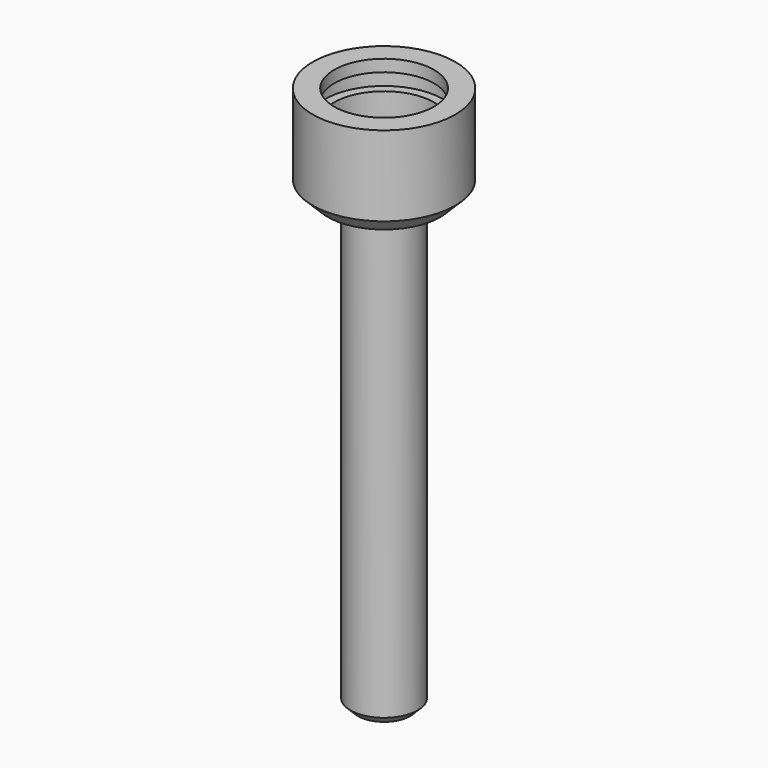
from build123d import *

# Parameters (mm, degrees)
F0_R     = 9.525
F1_DEPTH = 12.7
F2_R     = 6.6675
F3_DEPTH = 9.525
F4_W     = 1.1938
F4_H     = 2.2352
F7_SIZE  = 2
F8_R     = 4.485
F9_DEPTH = 60
F10_SIZE = 1


# Not quite as in the source:
# - the program builds the solid bodies; features that only make, move or delete a surface that nothing else refers to are left out


with BuildPart() as f1:
    # F0 (on Top) → F1 (new body)
    with BuildSketch(Plane.XY):
        Circle(F0_R)
    extrude(amount=F1_DEPTH)

    # F2 (on face) → F3 (cut)
    with BuildSketch(Plane.XY.offset(12.7)):
        Circle(F2_R)
    extrude(amount=-F3_DEPTH, mode=Mode.SUBTRACT)

    # F4 (on Front) → F5 (revolve, cut)
    with BuildSketch(Plane.XZ):
        with Locations((7.2644, 9.9949)):
            Rectangle(F4_W, F4_H)
    revolve(axis=Axis((0, 0, 19.0221574157), (0, 0, 1)), mode=Mode.SUBTRACT)

    # F7
    f7_edges = [f1.edges().sort_by_distance(p)[0] for p in [
        (-9.525, 0, 0),
    ]]
    chamfer(f7_edges, length=F7_SIZE)

    # F8 (on face) → F9 (join)
    with BuildSketch(Plane(origin=(0, 0, 0), x_dir=(1, 0, 0), z_dir=(0, 0, -1))):
        Circle(F8_R)
    extrude(amount=F9_DEPTH)

    # F10
    f10_edges = [f1.edges().sort_by_distance(p)[0] for p in [
        (-4.485, 0, -60),
    ]]
    chamfer(f10_edges, length=F10_SIZE)


solid = f1.part
